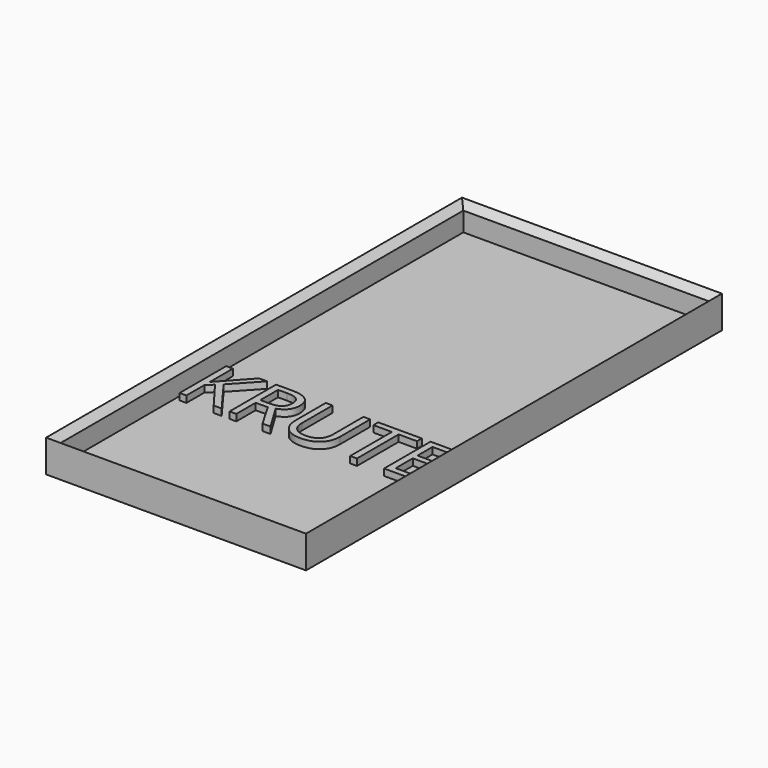
from build123d import *

# Parameters (mm, degrees)
F0_W         = 100
F0_H         = 200
F1_DEPTH     = 15
F2_T         = -2.54
F3_TEXT_SIZE = 31.2934800687
F4_DEPTH     = 2.54
F5_T1_DEPTH  = 194.92
F5_T3_DEPTH  = 94.92
F5_T9_DEPTH  = 207.9841495789
F5_T15_DEPTH = 107.9841495789
F5_T24_DEPTH = 207.9841495789
F5_T30_DEPTH = 107.9841495789
F5_T39_DEPTH = 207.9841495789
F5_T45_DEPTH = 107.9841495789
F5_T54_DEPTH = 107.9841495789
F5_T60_DEPTH = 207.9841495789


# Not quite as in the source:
# - a fillet or chamfer that OpenCascade refuses, or shapes differently, is made with other operations: its cross-section is extruded or revolved along the edge and cut away or added
# - Text() gives the source's letters only with a copy of the font that has no kerning and outlines rounded to 1/6400 em; it was checked with that copy


with BuildPart() as f1:
    # F0 (on Top) → F1 (new body)
    with BuildSketch(Plane.XY):
        with Locations((0.6390567869, 18.6407440308)):
            Rectangle(F0_W, F0_H)
    extrude(amount=F1_DEPTH)

    # F2
    f2_openings = [f1.faces().sort_by_distance(p)[0] for p in [
        (0.639057, 18.640744, 15),
    ]]
    offset(amount=F2_T, openings=f2_openings)

    # F3 (on face) → F4 (join)
    with BuildSketch(Plane.XY.offset(2.54)):
        with Locations((-48.0990567869, -22.5313056495)):
            Text('KRUTE', F3_TEXT_SIZE, font='Open Sans', text_align=(TextAlign.LEFT, TextAlign.BOTTOM))
    extrude(amount=F4_DEPTH)

    # F5: chamfer of 5.08 on 4 edges, made by hand

    # F5_s2 → F5_t1 (cut)
    with BuildSketch(Plane.XZ.offset(-116.1007440308)):
        Polygon((-51.9009432131, 15), (-46.8209432131, 9.92), (-46.8209432131, 15), align=None)
        Polygon((53.1790567869, 15), (48.0990567869, 9.92), (48.0990567869, 15), align=None)
    extrude(amount=F5_T1_DEPTH, mode=Mode.SUBTRACT)

    # F5_s4 → F5_t3 (cut)
    with BuildSketch(Plane.YZ.offset(-46.8209432131)):
        Polygon((-83.8992559692, 15), (-78.8192559692, 9.92), (-78.8192559692, 15), align=None)
        Polygon((121.1807440308, 15), (116.1007440308, 9.92), (116.1007440308, 15), align=None)
    extrude(amount=F5_T3_DEPTH, mode=Mode.SUBTRACT)


with BuildPart() as f5_tool7:
    # F5_s8 → F5_t9 (new body)
    with BuildSketch(Plane.XZ.offset(-129.1648936097)):
        Polygon((-51.9009432131, 15), (-46.8209432131, 9.92), (-46.8209432131, 15), align=None)
    extrude(amount=F5_T9_DEPTH)

    split(bisect_by=Plane.YZ.offset(-49.3609432131), keep=Keep.TOP)

    split(bisect_by=Plane.XZ.offset(-118.6407440308), keep=Keep.TOP)

    split(bisect_by=Plane.XZ.offset(-116.1007440308), keep=Keep.BOTTOM)


with BuildPart() as f5_tool13:
    # F5_s14 → F5_t15 (new body)
    with BuildSketch(Plane.YZ.offset(48.0990567869)):
        Polygon((121.1807440308, 15), (116.1007440308, 9.92), (116.1007440308, 15), align=None)
    extrude(amount=-F5_T15_DEPTH)

    split(bisect_by=Plane.YZ.offset(-49.3609432131), keep=Keep.TOP)

    split(bisect_by=Plane.XZ.offset(-118.6407440308), keep=Keep.TOP)

    split(bisect_by=Plane.YZ.offset(-46.8209432131), keep=Keep.BOTTOM)


with BuildPart() as f5_tool7_1:
    add(f5_tool7.part)

    # F5_t19: intersect F5_tool13
    add(f5_tool13.part, mode=Mode.INTERSECT)


with BuildPart() as f1_1:
    add(f1.part)

    # F5_t5: cut F5_tool7
    add(f5_tool7_1.part, mode=Mode.SUBTRACT)


with BuildPart() as f5_tool22:
    # F5_s23 → F5_t24 (new body)
    with BuildSketch(Plane.XZ.offset(-116.1007440308)):
        Polygon((-51.9009432131, 15), (-46.8209432131, 9.92), (-46.8209432131, 15), align=None)
    extrude(amount=F5_T24_DEPTH)

    split(bisect_by=Plane.YZ.offset(-49.3609432131), keep=Keep.TOP)

    split(bisect_by=Plane.XZ.offset(81.3592559692), keep=Keep.BOTTOM)

    split(bisect_by=Plane.XZ.offset(78.8192559692), keep=Keep.TOP)


with BuildPart() as f5_tool28:
    # F5_s29 → F5_t30 (new body)
    with BuildSketch(Plane.YZ.offset(-59.885092792)):
        Polygon((-83.8992559692, 15), (-78.8192559692, 9.92), (-78.8192559692, 15), align=None)
    extrude(amount=F5_T30_DEPTH)

    split(bisect_by=Plane.YZ.offset(-49.3609432131), keep=Keep.TOP)

    split(bisect_by=Plane.XZ.offset(81.3592559692), keep=Keep.BOTTOM)

    split(bisect_by=Plane.YZ.offset(-46.8209432131), keep=Keep.BOTTOM)


with BuildPart() as f5_tool22_1:
    add(f5_tool22.part)

    # F5_t34: intersect F5_tool28
    add(f5_tool28.part, mode=Mode.INTERSECT)


with BuildPart() as f1_2:
    add(f1_1.part)

    # F5_t20: cut F5_tool22
    add(f5_tool22_1.part, mode=Mode.SUBTRACT)


with BuildPart() as f5_tool37:
    # F5_s38 → F5_t39 (new body)
    with BuildSketch(Plane.XZ.offset(91.8834055481)):
        Polygon((53.1790567869, 15), (48.0990567869, 9.92), (48.0990567869, 15), align=None)
    extrude(amount=-F5_T39_DEPTH)

    split(bisect_by=Plane.XZ.offset(81.3592559692), keep=Keep.BOTTOM)

    split(bisect_by=Plane.YZ.offset(50.6390567869), keep=Keep.BOTTOM)

    split(bisect_by=Plane.XZ.offset(78.8192559692), keep=Keep.TOP)


with BuildPart() as f5_tool43:
    # F5_s44 → F5_t45 (new body)
    with BuildSketch(Plane.YZ.offset(-46.8209432131)):
        Polygon((-83.8992559692, 15), (-78.8192559692, 9.92), (-78.8192559692, 15), align=None)
    extrude(amount=F5_T45_DEPTH)

    split(bisect_by=Plane.XZ.offset(81.3592559692), keep=Keep.BOTTOM)

    split(bisect_by=Plane.YZ.offset(50.6390567869), keep=Keep.BOTTOM)

    split(bisect_by=Plane.YZ.offset(48.0990567869), keep=Keep.TOP)


with BuildPart() as f5_tool37_1:
    add(f5_tool37.part)

    # F5_t49: intersect F5_tool43
    add(f5_tool43.part, mode=Mode.INTERSECT)


with BuildPart() as f1_3:
    add(f1_2.part)

    # F5_t35: cut F5_tool37
    add(f5_tool37_1.part, mode=Mode.SUBTRACT)


with BuildPart() as f5_tool52:
    # F5_s53 → F5_t54 (new body)
    with BuildSketch(Plane.YZ.offset(61.1632063658)):
        Polygon((121.1807440308, 15), (116.1007440308, 9.92), (116.1007440308, 15), align=None)
    extrude(amount=-F5_T54_DEPTH)

    split(bisect_by=Plane.XZ.offset(-118.6407440308), keep=Keep.TOP)

    split(bisect_by=Plane.YZ.offset(50.6390567869), keep=Keep.BOTTOM)

    split(bisect_by=Plane.YZ.offset(48.0990567869), keep=Keep.TOP)


with BuildPart() as f5_tool58:
    # F5_s59 → F5_t60 (new body)
    with BuildSketch(Plane.XZ.offset(78.8192559692)):
        Polygon((53.1790567869, 15), (48.0990567869, 9.92), (48.0990567869, 15), align=None)
    extrude(amount=-F5_T60_DEPTH)

    split(bisect_by=Plane.XZ.offset(-118.6407440308), keep=Keep.TOP)

    split(bisect_by=Plane.YZ.offset(50.6390567869), keep=Keep.BOTTOM)

    split(bisect_by=Plane.XZ.offset(-116.1007440308), keep=Keep.BOTTOM)


with BuildPart() as f5_tool52_1:
    add(f5_tool52.part)

    # F5_t64: intersect F5_tool58
    add(f5_tool58.part, mode=Mode.INTERSECT)


with BuildPart() as f1_4:
    add(f1_3.part)

    # F5_t50: cut F5_tool52
    add(f5_tool52_1.part, mode=Mode.SUBTRACT)


solid = f1_4.part
